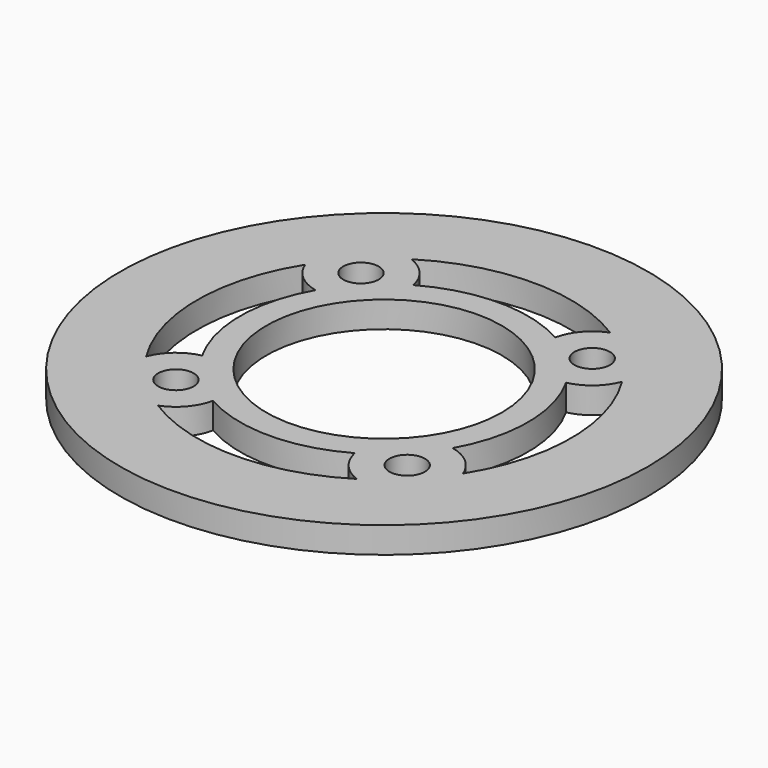
from build123d import *

# Parameters (mm, degrees)
F0_R            = 32.0294
F0_R_2          = 2.15265
F0_R_3          = 14.2875
F1_DEPTH        = 3.175
F3_DEPTH        = 3.175
F3_COPIES_COUNT = 4


# Not quite as in the source:
# - a pattern or mirror of a feature is missing from the dataset's text; its kind, count and spacing are read off the source's solid


with BuildPart() as f1:
    # F0 (on Top) → F1 (new body)
    with BuildSketch(Plane.XY):
        Circle(F0_R)
        with Locations((-14.0316501892, -14.0316501892)):
            Circle(F0_R_2, mode=Mode.SUBTRACT)
        with Locations((14.0316501892, -14.0316501892)):
            Circle(F0_R_2, mode=Mode.SUBTRACT)
        with Locations((-14.0316501892, 14.0316501892)):
            Circle(F0_R_2, mode=Mode.SUBTRACT)
        Circle(F0_R_3, mode=Mode.SUBTRACT)
        with Locations((14.0316501892, 14.0316501892)):
            Circle(F0_R_2, mode=Mode.SUBTRACT)
    extrude(amount=F1_DEPTH)

    # F2 (on face) → F3 (cut, through all)
    with BuildSketch(Plane.XY.offset(3.175)):
        with BuildLine():
            ThreePointArc((-12.0590655259, 19.2259570543), (-9.8169566913, 17.6521850643), (-8.599282572, 15.1983961488))
            ThreePointArc((-8.599282572, 15.1983961488), (0, 17.4625), (8.599282572, 15.1983961488))
            ThreePointArc((8.599282572, 15.1983961488), (9.8169566913, 17.6521850643), (12.0590655259, 19.2259570543))
            ThreePointArc((12.0590655259, 19.2259570543), (0, 22.6949), (-12.0590655259, 19.2259570543))
        make_face()
    f3 = extrude(amount=-F3_DEPTH, mode=Mode.SUBTRACT)

    # F3_copies: F3 ×4 about axis
    f3_copies_axis = Axis((0, 0, 0), (0, 0, 1))
    for i in range(1, F3_COPIES_COUNT):
        add(f3.rotate(f3_copies_axis, i * 360 / F3_COPIES_COUNT), mode=Mode.SUBTRACT)


solid = f1.part
